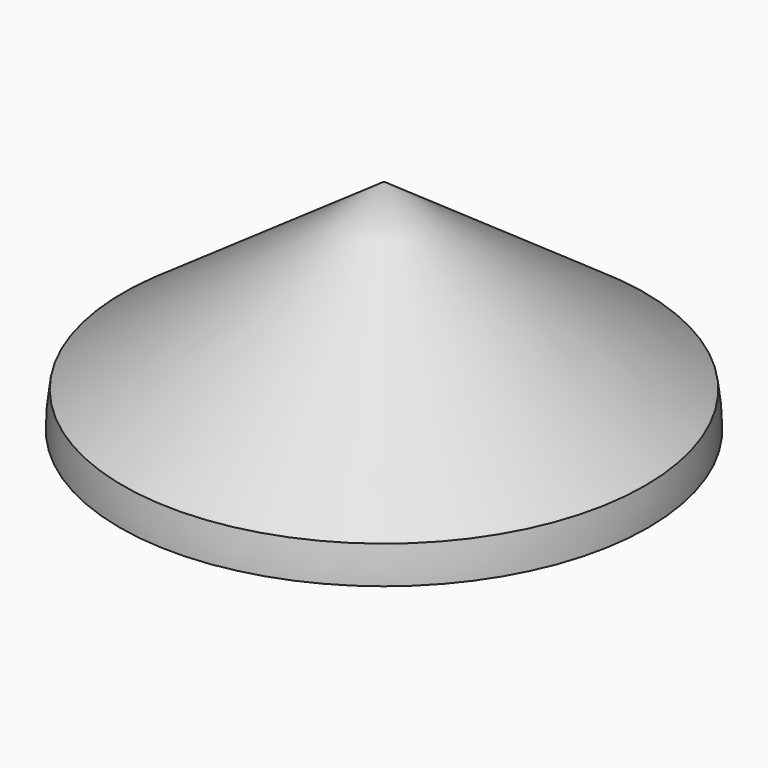
from build123d import *


# Not quite as in the source:
# - the dataset's text gives a spline's control points without its knots; the knots are read off the source's solid


with BuildPart() as f1:
    # F0 (on Front) → F1 (revolve)
    with BuildSketch(Plane.XZ):
        with BuildLine():
            Line((-15015.1641677809, -9485.9644285342), (14113.7343711964, -9485.9644285342))
            add(Edge.make_bspline(
                [(14113.7343711964, -9485.9644285342), (14111.0684335143, -9470.3167211759), (14108.3867099418, -9454.671133503), (14105.6892044539, -9439.0276907001)],
                knots=[6.4346155813, 6.4346155813, 6.4346155813, 6.4346155813, 6.4364231918, 6.4364231918, 6.4364231918, 6.4364231918], degree=3))
            Line((14105.6892044538, -9439.0276907002), (-15015.1641677809, 10951.6133596381))
            Line((-15015.1641677809, 10951.6133596381), (-15015.1641677809, -9485.9644285342))
        make_face()
        with BuildLine():
            Line((-15015.1641677809, -13448.3644285342), (14449.3753730529, -13448.3644285342))
            add(Edge.make_bspline(
                [(14449.3753730529, -13448.3644285342), (14449.3753730529, -12749.9900368383), (14418.2604711201, -12051.6160368424), (14300.3029043107, -10729.9828852019), (14219.4237908412, -10106.3079274051), (14113.7343711964, -9485.9644285342)],
                knots=[6.283185, 6.283185, 6.283185, 6.283185, 6.362954, 6.362954, 6.4346155813, 6.4346155813, 6.4346155813, 6.4346155813], degree=3))
            Line((14113.7343711964, -9485.9644285342), (-15015.1641677809, -9485.9644285342))
            Line((-15015.1641677809, -9485.9644285342), (-15015.1641677809, -13448.3644285342))
        make_face()
    revolve(axis=Axis((-15015.1641677809, 0, -1248.375534448), (0, 0, 1)))


solid = f1.part
